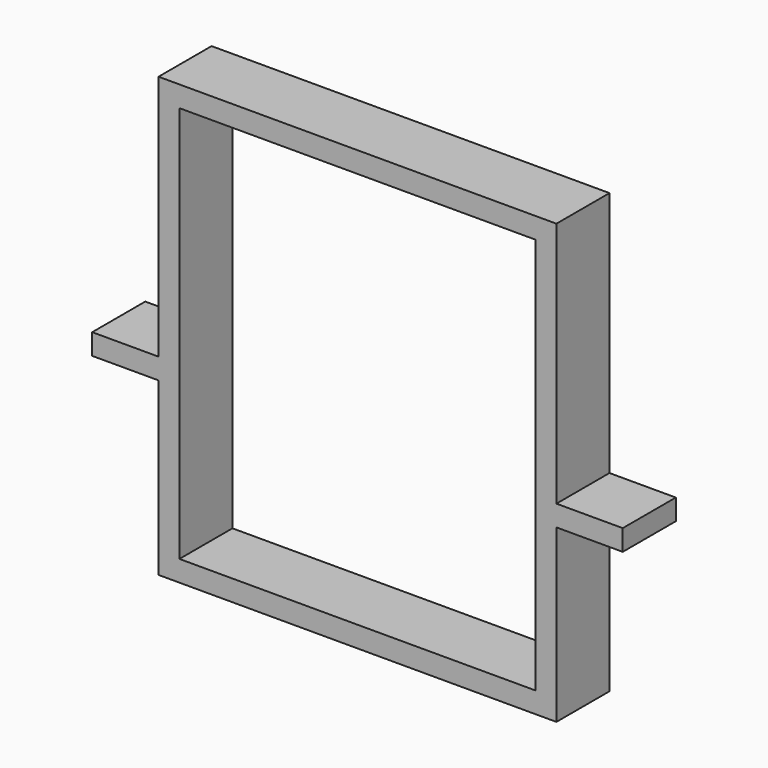
from build123d import *

# Parameters (mm, degrees)
F1_DEPTH = 6.35


# Not quite as in the source:
# - a length typed as a fraction of an inch, garbled in the dataset ("3 / 203.2 mm" for 3/8 in), is restored


with BuildPart() as f1:
    # F0 (on Front) → F1 (new body)
    with BuildSketch(Plane.XZ):
        Polygon((-25.4000015863, 18.4), (-25.4, 16.4), (-19.05, 16.4), (-19.05, 0), (0, 0), (0, 2), (-17.05, 2), (-17.05, 40), (0, 40), (0, 42), (-19.05, 42), (-19.05, 18.4), align=None)
    extrude(amount=F1_DEPTH)

    # F2: F1 across plane


with BuildPart() as f1_1:
    add(f1.part)
    add(f1.part.mirror(Plane.YZ))


solid = f1_1.part
